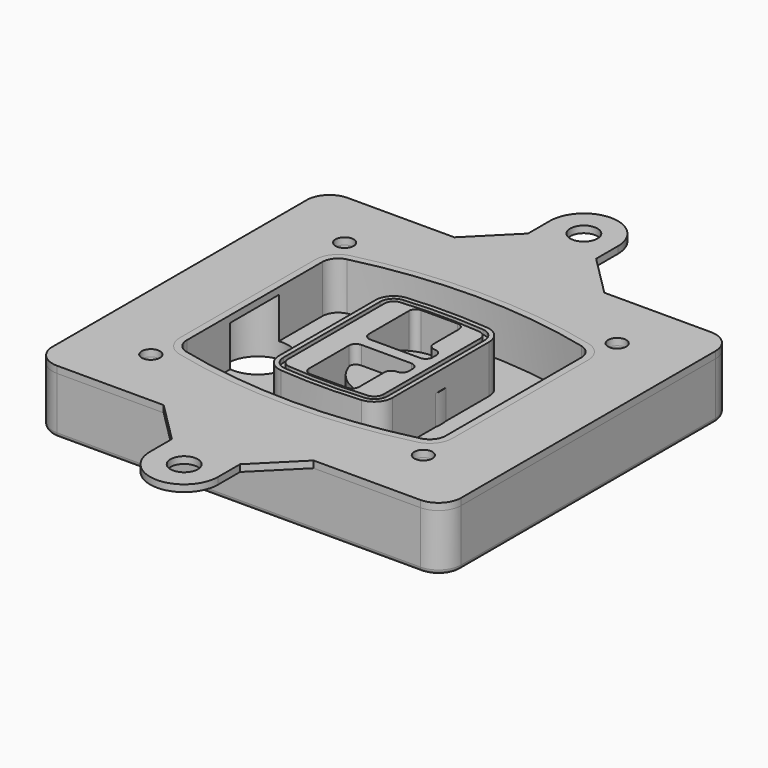
from build123d import *

# Parameters (mm, degrees)
F0_R      = 4
F1_DEPTH  = 25
F2_DEPTH  = 3
F3_DEPTH  = 18
F5_DEPTH  = 21
F6_DEPTH  = 2
F8_DEPTH  = 20
F9_DEPTH  = 16
F10_DEPTH = 25
F7_R      = 6
F7_R_2    = 4
F11_DEPTH = 6
F13_DEPTH = 9
F15_R     = 2
F16_R     = 4
F16_R_2   = 6
F17_DEPTH = 3


# Not quite as in the source:
# - a feature of the source that left no trace in its solid (it failed there, or was rolled back) is left out
# - a feature names something its author has since deleted; it is built from what else it names


with BuildPart() as f1:
    # F0 (on Top) → F1 (new body)
    with BuildSketch(Plane.XY):
        with BuildLine():
            ThreePointArc((-90, -70), (-87.0710678119, -77.0710678119), (-80, -80))
            Line((-80, -80), (80, -80))
            ThreePointArc((80, -80), (87.0710678119, -77.0710678119), (90, -70))
            Line((90, -70), (90, 70))
            ThreePointArc((90, 70), (87.0710678119, 77.0710678119), (80, 80))
            Line((80, 80), (-80, 80))
            ThreePointArc((-80, 80), (-87.0710678119, 77.0710678119), (-90, 70))
            Line((-90, 70), (-90, -70))
        make_face()
        with Locations((-60, -53.3333333333)):
            Circle(F0_R, mode=Mode.SUBTRACT)
        with Locations((60, -53.3333333333)):
            Circle(F0_R, mode=Mode.SUBTRACT)
        with Locations((-60, 53.3333333333)):
            Circle(F0_R, mode=Mode.SUBTRACT)
        with BuildLine():
            ThreePointArc((-64, 37.2990447398), (-61.0143011354, 45.9411029726), (-53.3306899286, 50.8970778549))
            ThreePointArc((-53.3306899286, 50.8970778549), (0, 57.3333333333), (53.3306899286, 50.8970778549))
            ThreePointArc((53.3306899286, 50.8970778549), (61.0143011354, 45.9411029726), (64, 37.2990447398))
            Line((64, 37.2990447398), (64, -37.2990447398))
            ThreePointArc((64, -37.2990447398), (61.0143011354, -45.9411029726), (53.3306899286, -50.8970778549))
            ThreePointArc((53.3306899286, -50.8970778549), (0, -57.3333333333), (-53.3306899286, -50.8970778549))
            ThreePointArc((-53.3306899286, -50.8970778549), (-61.0143011354, -45.9411029726), (-64, -37.2990447398))
            Line((-64, -37.2990447398), (-64, 37.2990447398))
        make_face(mode=Mode.SUBTRACT)
        with Locations((60, 53.3333333333)):
            Circle(F0_R, mode=Mode.SUBTRACT)
        with BuildLine():
            ThreePointArc((53.3306899286, 50.8970778549), (0, 57.3333333333), (-53.3306899286, 50.8970778549))
            ThreePointArc((-53.3306899286, 50.8970778549), (-61.0143011354, 45.9411029726), (-64, 37.2990447398))
            Line((-64, 37.2990447398), (-64, -37.2990447398))
            ThreePointArc((-64, -37.2990447398), (-61.0143011354, -45.9411029726), (-53.3306899286, -50.8970778549))
            ThreePointArc((-53.3306899286, -50.8970778549), (0, -57.3333333333), (53.3306899286, -50.8970778549))
            ThreePointArc((53.3306899286, -50.8970778549), (61.0143011354, -45.9411029726), (64, -37.2990447398))
            Line((64, -37.2990447398), (64, 37.2990447398))
            ThreePointArc((64, 37.2990447398), (61.0143011354, 45.9411029726), (53.3306899286, 50.8970778549))
        make_face()
        with BuildLine():
            Line((-60, -37.2990447398), (-60, 37.2990447398))
            ThreePointArc((-60, 37.2990447398), (-57.8673579538, 43.4719434775), (-52.3790642347, 47.0119255363))
            ThreePointArc((-52.3790642347, 47.0119255363), (0, 53.3333333333), (52.3790642347, 47.0119255363))
            ThreePointArc((52.3790642347, 47.0119255363), (57.8673579538, 43.4719434775), (60, 37.2990447398))
            Line((60, 37.2990447398), (60, -37.2990447398))
            ThreePointArc((60, -37.2990447398), (57.8673579538, -43.4719434775), (52.3790642347, -47.0119255363))
            ThreePointArc((52.3790642347, -47.0119255363), (0, -53.3333333333), (-52.3790642347, -47.0119255363))
            ThreePointArc((-52.3790642347, -47.0119255363), (-57.8673579538, -43.4719434775), (-60, -37.2990447398))
        make_face(mode=Mode.SUBTRACT)
        with BuildLine():
            ThreePointArc((-52.3790642347, 47.0119255363), (-57.8673579538, 43.4719434775), (-60, 37.2990447398))
            Line((-60, 37.2990447398), (-60, -37.2990447398))
            ThreePointArc((-60, -37.2990447398), (-57.8673579538, -43.4719434775), (-52.3790642347, -47.0119255363))
            ThreePointArc((-52.3790642347, -47.0119255363), (0, -53.3333333333), (52.3790642347, -47.0119255363))
            ThreePointArc((52.3790642347, -47.0119255363), (57.8673579538, -43.4719434775), (60, -37.2990447398))
            Line((60, -37.2990447398), (60, 37.2990447398))
            ThreePointArc((60, 37.2990447398), (57.8673579538, 43.4719434775), (52.3790642347, 47.0119255363))
            ThreePointArc((52.3790642347, 47.0119255363), (0, 53.3333333333), (-52.3790642347, 47.0119255363))
        make_face()
        with BuildLine():
            ThreePointArc((51.6653449643, 44.0980612973), (55.5071505677, 41.6200738562), (57, 37.2990447398))
            Line((57, 37.2990447398), (57, -37.2990447398))
            ThreePointArc((57, -37.2990447398), (55.5071505677, -41.6200738562), (51.6653449643, -44.0980612973))
            ThreePointArc((51.6653449643, -44.0980612973), (0, -50.3333333333), (-51.6653449643, -44.0980612973))
            ThreePointArc((-51.6653449643, -44.0980612973), (-55.5071505677, -41.6200738562), (-57, -37.2990447398))
            Line((-57, -37.2990447398), (-57, 37.2990447398))
            ThreePointArc((-57, 37.2990447398), (-55.5071505677, 41.6200738562), (-51.6653449643, 44.0980612973))
            ThreePointArc((-51.6653449643, 44.0980612973), (0, 50.3333333333), (51.6653449643, 44.0980612973))
        make_face(mode=Mode.SUBTRACT)
        with BuildLine():
            Line((57, -37.2990447398), (57, 37.2990447398))
            ThreePointArc((57, 37.2990447398), (55.5071505677, 41.6200738562), (51.6653449643, 44.0980612973))
            ThreePointArc((51.6653449643, 44.0980612973), (0, 50.3333333333), (-51.6653449643, 44.0980612973))
            ThreePointArc((-51.6653449643, 44.0980612973), (-55.5071505677, 41.6200738562), (-57, 37.2990447398))
            Line((-57, 37.2990447398), (-57, -37.2990447398))
            ThreePointArc((-57, -37.2990447398), (-55.5071505677, -41.6200738562), (-51.6653449643, -44.0980612973))
            ThreePointArc((-51.6653449643, -44.0980612973), (0, -50.3333333333), (51.6653449643, -44.0980612973))
            ThreePointArc((51.6653449643, -44.0980612973), (55.5071505677, -41.6200738562), (57, -37.2990447398))
        make_face()
    extrude(amount=-F1_DEPTH)

    # F0 (on Top) → F2 (join)
    with BuildSketch(Plane.XY):
        with BuildLine():
            ThreePointArc((-52.3790642347, 47.0119255363), (-57.8673579538, 43.4719434775), (-60, 37.2990447398))
            Line((-60, 37.2990447398), (-60, -37.2990447398))
            ThreePointArc((-60, -37.2990447398), (-57.8673579538, -43.4719434775), (-52.3790642347, -47.0119255363))
            ThreePointArc((-52.3790642347, -47.0119255363), (0, -53.3333333333), (52.3790642347, -47.0119255363))
            ThreePointArc((52.3790642347, -47.0119255363), (57.8673579538, -43.4719434775), (60, -37.2990447398))
            Line((60, -37.2990447398), (60, 37.2990447398))
            ThreePointArc((60, 37.2990447398), (57.8673579538, 43.4719434775), (52.3790642347, 47.0119255363))
            ThreePointArc((52.3790642347, 47.0119255363), (0, 53.3333333333), (-52.3790642347, 47.0119255363))
        make_face()
        with BuildLine():
            ThreePointArc((51.6653449643, 44.0980612973), (55.5071505677, 41.6200738562), (57, 37.2990447398))
            Line((57, 37.2990447398), (57, -37.2990447398))
            ThreePointArc((57, -37.2990447398), (55.5071505677, -41.6200738562), (51.6653449643, -44.0980612973))
            ThreePointArc((51.6653449643, -44.0980612973), (0, -50.3333333333), (-51.6653449643, -44.0980612973))
            ThreePointArc((-51.6653449643, -44.0980612973), (-55.5071505677, -41.6200738562), (-57, -37.2990447398))
            Line((-57, -37.2990447398), (-57, 37.2990447398))
            ThreePointArc((-57, 37.2990447398), (-55.5071505677, 41.6200738562), (-51.6653449643, 44.0980612973))
            ThreePointArc((-51.6653449643, 44.0980612973), (0, 50.3333333333), (51.6653449643, 44.0980612973))
        make_face(mode=Mode.SUBTRACT)
    extrude(amount=F2_DEPTH)

    # F0 (on Top) → F3 (cut)
    with BuildSketch(Plane.XY):
        with BuildLine():
            Line((57, -37.2990447398), (57, 37.2990447398))
            ThreePointArc((57, 37.2990447398), (55.5071505677, 41.6200738562), (51.6653449643, 44.0980612973))
            ThreePointArc((51.6653449643, 44.0980612973), (0, 50.3333333333), (-51.6653449643, 44.0980612973))
            ThreePointArc((-51.6653449643, 44.0980612973), (-55.5071505677, 41.6200738562), (-57, 37.2990447398))
            Line((-57, 37.2990447398), (-57, -37.2990447398))
            ThreePointArc((-57, -37.2990447398), (-55.5071505677, -41.6200738562), (-51.6653449643, -44.0980612973))
            ThreePointArc((-51.6653449643, -44.0980612973), (0, -50.3333333333), (51.6653449643, -44.0980612973))
            ThreePointArc((51.6653449643, -44.0980612973), (55.5071505677, -41.6200738562), (57, -37.2990447398))
        make_face()
    extrude(amount=-F3_DEPTH, mode=Mode.SUBTRACT)

    # F4 (on face) → F5 (join, through all)
    with BuildSketch(Plane.XY.offset(3)):
        with BuildLine():
            ThreePointArc((-25, -26.587695628), (-22.8992979869, -31.9912392117), (-17.7004291845, -34.5569740744))
            ThreePointArc((-17.7004291845, -34.5569740744), (0, -35.3333333333), (17.7004291845, -34.5569740744))
            ThreePointArc((17.7004291845, -34.5569740744), (22.8992979869, -31.9912392117), (25, -26.587695628))
            Line((25, -26.587695628), (25, 26.587695628))
            ThreePointArc((25, 26.587695628), (22.8992979869, 31.9912392117), (17.7004291845, 34.5569740744))
            ThreePointArc((17.7004291845, 34.5569740744), (0, 35.3333333333), (-17.7004291845, 34.5569740744))
            ThreePointArc((-17.7004291845, 34.5569740744), (-22.8992979869, 31.9912392117), (-25, 26.587695628))
            Line((-25, 26.587695628), (-25, -26.587695628))
        make_face()
        with BuildLine():
            ThreePointArc((17.5253218884, 32.5646544628), (21.4244734902, 30.6403533158), (23, 26.587695628))
            Line((23, 26.587695628), (23, -26.587695628))
            ThreePointArc((23, -26.587695628), (21.4244734902, -30.6403533158), (17.5253218884, -32.5646544628))
            ThreePointArc((17.5253218884, -32.5646544628), (0, -33.3333333333), (-17.5253218884, -32.5646544628))
            ThreePointArc((-17.5253218884, -32.5646544628), (-21.4244734902, -30.6403533158), (-23, -26.587695628))
            Line((-23, -26.587695628), (-23, 26.587695628))
            ThreePointArc((-23, 26.587695628), (-21.4244734902, 30.6403533158), (-17.5253218884, 32.5646544628))
            ThreePointArc((-17.5253218884, 32.5646544628), (0, 33.3333333333), (17.5253218884, 32.5646544628))
        make_face(mode=Mode.SUBTRACT)
        with BuildLine():
            Line((23, -26.587695628), (23, 26.587695628))
            ThreePointArc((23, 26.587695628), (21.4244734902, 30.6403533158), (17.5253218884, 32.5646544628))
            ThreePointArc((17.5253218884, 32.5646544628), (0, 33.3333333333), (-17.5253218884, 32.5646544628))
            ThreePointArc((-17.5253218884, 32.5646544628), (-21.4244734902, 30.6403533158), (-23, 26.587695628))
            Line((-23, 26.587695628), (-23, -26.587695628))
            ThreePointArc((-23, -26.587695628), (-21.4244734902, -30.6403533158), (-17.5253218884, -32.5646544628))
            ThreePointArc((-17.5253218884, -32.5646544628), (0, -33.3333333333), (17.5253218884, -32.5646544628))
            ThreePointArc((17.5253218884, -32.5646544628), (21.4244734902, -30.6403533158), (23, -26.587695628))
        make_face()
        with BuildLine():
            ThreePointArc((17.3502145923, 30.5723348512), (19.9496489934, 29.2894674198), (21, 26.587695628))
            Line((21, 26.587695628), (21, -26.587695628))
            ThreePointArc((21, -26.587695628), (19.9496489934, -29.2894674198), (17.3502145923, -30.5723348512))
            ThreePointArc((17.3502145923, -30.5723348512), (0, -31.3333333333), (-17.3502145923, -30.5723348512))
            ThreePointArc((-17.3502145923, -30.5723348512), (-19.9496489934, -29.2894674198), (-21, -26.587695628))
            Line((-21, -26.587695628), (-21, 26.587695628))
            ThreePointArc((-21, 26.587695628), (-19.9496489934, 29.2894674198), (-17.3502145923, 30.5723348512))
            ThreePointArc((-17.3502145923, 30.5723348512), (0, 31.3333333333), (17.3502145923, 30.5723348512))
        make_face(mode=Mode.SUBTRACT)
        with BuildLine():
            Line((21, -26.587695628), (21, 26.587695628))
            ThreePointArc((21, 26.587695628), (19.9496489934, 29.2894674198), (17.3502145923, 30.5723348512))
            ThreePointArc((17.3502145923, 30.5723348512), (0, 31.3333333333), (-17.3502145923, 30.5723348512))
            ThreePointArc((-17.3502145923, 30.5723348512), (-19.9496489934, 29.2894674198), (-21, 26.587695628))
            Line((-21, 26.587695628), (-21, -26.587695628))
            ThreePointArc((-21, -26.587695628), (-19.9496489934, -29.2894674198), (-17.3502145923, -30.5723348512))
            ThreePointArc((-17.3502145923, -30.5723348512), (0, -31.3333333333), (17.3502145923, -30.5723348512))
            ThreePointArc((17.3502145923, -30.5723348512), (19.9496489934, -29.2894674198), (21, -26.587695628))
        make_face()
        with BuildLine():
            Line((-8, -2.5), (14, -2.5))
            ThreePointArc((14, -2.5), (16.1213203436, -3.3786796564), (17, -5.5))
            Line((17, -5.5), (17, -7.5))
            ThreePointArc((17, -7.5), (16.1213203436, -9.6213203436), (14, -10.5))
            ThreePointArc((14, -10.5), (11.8786796564, -11.3786796564), (11, -13.5))
            Line((11, -13.5), (11, -27.5))
            ThreePointArc((11, -27.5), (10.1213203436, -29.6213203436), (8, -30.5))
            Line((8, -30.5), (-8, -30.5))
            ThreePointArc((-8, -30.5), (-10.1213203436, -29.6213203436), (-11, -27.5))
            Line((-11, -27.5), (-11, -5.5))
            ThreePointArc((-11, -5.5), (-10.1213203436, -3.3786796564), (-8, -2.5))
        make_face(mode=Mode.SUBTRACT)
        with BuildLine():
            ThreePointArc((-8, 2.5), (-10.1213203436, 3.3786796564), (-11, 5.5))
            Line((-11, 5.5), (-11, 27.5))
            ThreePointArc((-11, 27.5), (-10.1213203436, 29.6213203436), (-8, 30.5))
            Line((-8, 30.5), (8, 30.5))
            ThreePointArc((8, 30.5), (10.1213203436, 29.6213203436), (11, 27.5))
            Line((11, 27.5), (11, 13.5))
            ThreePointArc((11, 13.5), (11.8786796564, 11.3786796564), (14, 10.5))
            ThreePointArc((14, 10.5), (16.1213203436, 9.6213203436), (17, 7.5))
            Line((17, 7.5), (17, 5.5))
            ThreePointArc((17, 5.5), (16.1213203436, 3.3786796564), (14, 2.5))
            Line((14, 2.5), (-8, 2.5))
        make_face(mode=Mode.SUBTRACT)
    extrude(amount=-F5_DEPTH)

    # F4 (on face) → F6 (cut)
    with BuildSketch(Plane.XY.offset(3)):
        with BuildLine():
            Line((23, -26.587695628), (23, 26.587695628))
            ThreePointArc((23, 26.587695628), (21.4244734902, 30.6403533158), (17.5253218884, 32.5646544628))
            ThreePointArc((17.5253218884, 32.5646544628), (0, 33.3333333333), (-17.5253218884, 32.5646544628))
            ThreePointArc((-17.5253218884, 32.5646544628), (-21.4244734902, 30.6403533158), (-23, 26.587695628))
            Line((-23, 26.587695628), (-23, -26.587695628))
            ThreePointArc((-23, -26.587695628), (-21.4244734902, -30.6403533158), (-17.5253218884, -32.5646544628))
            ThreePointArc((-17.5253218884, -32.5646544628), (0, -33.3333333333), (17.5253218884, -32.5646544628))
            ThreePointArc((17.5253218884, -32.5646544628), (21.4244734902, -30.6403533158), (23, -26.587695628))
        make_face()
        with BuildLine():
            ThreePointArc((17.3502145923, 30.5723348512), (19.9496489934, 29.2894674198), (21, 26.587695628))
            Line((21, 26.587695628), (21, -26.587695628))
            ThreePointArc((21, -26.587695628), (19.9496489934, -29.2894674198), (17.3502145923, -30.5723348512))
            ThreePointArc((17.3502145923, -30.5723348512), (0, -31.3333333333), (-17.3502145923, -30.5723348512))
            ThreePointArc((-17.3502145923, -30.5723348512), (-19.9496489934, -29.2894674198), (-21, -26.587695628))
            Line((-21, -26.587695628), (-21, 26.587695628))
            ThreePointArc((-21, 26.587695628), (-19.9496489934, 29.2894674198), (-17.3502145923, 30.5723348512))
            ThreePointArc((-17.3502145923, 30.5723348512), (0, 31.3333333333), (17.3502145923, 30.5723348512))
        make_face(mode=Mode.SUBTRACT)
    extrude(amount=-F6_DEPTH, mode=Mode.SUBTRACT)

    # F7 (on face) → F8 (join)
    with BuildSketch(Plane(origin=(0, 0, -25), x_dir=(1, 0, 0), z_dir=(0, 0, -1))):
        with BuildLine():
            ThreePointArc((-6.71157564, 0), (6.7567035675, 13.4682792075), (20.224982775, 0))
            Line((20.224982775, 0), (25.224982775, 0))
            ThreePointArc((25.224982775, 0), (6.7567035675, 18.4682792075), (-11.71157564, 0))
            Line((-11.71157564, 0), (-6.71157564, 0))
        make_face()
        with BuildLine():
            Line((-6.71157564, 0), (20.224982775, 0))
            ThreePointArc((20.224982775, 0), (6.7567035675, 13.4682792075), (-6.71157564, 0))
        make_face()
        with BuildLine():
            ThreePointArc((-6.71157564, 0), (6.7567035675, -13.4682792075), (20.224982775, 0))
            Line((20.224982775, 0), (-6.71157564, 0))
        make_face()
        with BuildLine():
            Line((25.224982775, 0), (20.224982775, 0))
            ThreePointArc((20.224982775, 0), (6.7567035675, -13.4682792075), (-6.71157564, 0))
            Line((-6.71157564, 0), (-11.71157564, 0))
            ThreePointArc((-11.71157564, 0), (6.7567035675, -18.4682792075), (25.224982775, 0))
        make_face()
    extrude(amount=-F8_DEPTH)

    # F7 (on face) → F9 (cut)
    with BuildSketch(Plane(origin=(0, 0, -25), x_dir=(1, 0, 0), z_dir=(0, 0, -1))):
        with BuildLine():
            Line((-6.71157564, 0), (20.224982775, 0))
            ThreePointArc((20.224982775, 0), (6.7567035675, 13.4682792075), (-6.71157564, 0))
        make_face()
        with BuildLine():
            ThreePointArc((-6.71157564, 0), (6.7567035675, -13.4682792075), (20.224982775, 0))
            Line((20.224982775, 0), (-6.71157564, 0))
        make_face()
    extrude(amount=-F9_DEPTH, mode=Mode.SUBTRACT)

    # F7 (on face) → F10 (cut)
    with BuildSketch(Plane(origin=(0, 0, -25), x_dir=(1, 0, 0), z_dir=(0, 0, -1))):
        with BuildLine():
            Line((-69.0318229325, 0), (-42.0952645175, 0))
            ThreePointArc((-42.0952645175, 0), (-55.563543725, 13.4682792075), (-69.0318229325, 0))
        make_face()
        with BuildLine():
            ThreePointArc((-69.0318229325, 0), (-55.563543725, -13.4682792075), (-42.0952645175, 0))
            Line((-42.0952645175, 0), (-69.0318229325, 0))
        make_face()
    extrude(amount=-F10_DEPTH, mode=Mode.SUBTRACT)

    # F7 (on face) → F11 (cut)
    with BuildSketch(Plane(origin=(0, 0, -25), x_dir=(1, 0, 0), z_dir=(0, 0, -1))):
        with Locations((60, -53.3333333333)):
            Circle(F7_R)
        with Locations((60, -53.3333333333)):
            Circle(F7_R_2, mode=Mode.SUBTRACT)
        with Locations((-60, -53.3333333333)):
            Circle(F7_R)
        with Locations((-60, -53.3333333333)):
            Circle(F7_R_2, mode=Mode.SUBTRACT)
        with Locations((-60, 53.3333333333)):
            Circle(F7_R)
        with Locations((-60, 53.3333333333)):
            Circle(F7_R_2, mode=Mode.SUBTRACT)
        with Locations((60, 53.3333333333)):
            Circle(F7_R)
        with Locations((60, 53.3333333333)):
            Circle(F7_R_2, mode=Mode.SUBTRACT)
    extrude(amount=-F11_DEPTH, mode=Mode.SUBTRACT)

    # F12 (on face) → F13 (cut, through all)
    with BuildSketch(Plane(origin=(0, 0, -9), x_dir=(1, 0, 0), z_dir=(0, 0, -1))):
        with BuildLine():
            ThreePointArc((20.224982775, 0), (20.1663399806, 1.2554664788), (19.9909222755, 2.5))
            Line((19.9909222755, 2.5), (14, 2.5))
            ThreePointArc((14, 2.5), (16.1213203436, 3.3786796564), (17, 5.5))
            Line((17, 5.5), (17, 7.5))
            ThreePointArc((17, 7.5), (16.1213203436, 9.6213203436), (14, 10.5))
            ThreePointArc((14, 10.5), (12.1627255951, 11.1284134507), (11.0951631559, 12.750384826))
            ThreePointArc((11.0951631559, 12.750384826), (11.0476113807, 12.7664660322), (11, 12.7823698976))
            Line((11, 12.7823698976), (11, -12.7823698976))
            ThreePointArc((11, -12.7823698976), (11.0476113807, -12.7664660322), (11.0951631559, -12.750384826))
            ThreePointArc((11.0951631559, -12.750384826), (12.1627255951, -11.1284134507), (14, -10.5))
            ThreePointArc((14, -10.5), (16.1213203436, -9.6213203436), (17, -7.5))
            Line((17, -7.5), (17, -5.5))
            ThreePointArc((17, -5.5), (16.1213203436, -3.3786796564), (14, -2.5))
            Line((14, -2.5), (19.9909222755, -2.5))
            ThreePointArc((19.9909222755, -2.5), (20.1663399806, -1.2554664788), (20.224982775, 0))
        make_face()
    extrude(amount=F13_DEPTH, mode=Mode.SUBTRACT)

    # F15
    f15_edges = [f1.edges().sort_by_distance(p)[0] for p in [
        (0, -80, -25),
        (-87.071068, -77.071068, -25),
        (-90, 0, -25),
        (-87.071068, 77.071068, -25),
        (87.071068, -77.071068, -25),
        (0, 80, -25),
        (90, 0, -25),
        (87.071068, 77.071068, -25),
    ]]
    fillet(f15_edges, radius=F15_R)


with BuildPart() as f17:
    # F16 (on face) → F17 (new body, through all)
    with BuildSketch(Plane.XY):
        with BuildLine():
            Line((-33, 80), (-80, 80))
            ThreePointArc((-80, 80), (-87.0710678119, 77.0710678119), (-90, 70))
            Line((-90, 70), (-90, -70))
            ThreePointArc((-90, -70), (-87.0710678119, -77.0710678119), (-80, -80))
            Line((-80, -80), (-33, -80))
            Line((-33, -80), (33, -80))
            Line((33, -80), (80, -80))
            ThreePointArc((80, -80), (87.0710678119, -77.0710678119), (90, -70))
            Line((90, -70), (90, 70))
            ThreePointArc((90, 70), (87.0710678119, 77.0710678119), (80, 80))
            Line((80, 80), (33, 80))
            Line((33, 80), (-33, 80))
        make_face()
        with Locations((-60, -53.3333333333)):
            Circle(F16_R, mode=Mode.SUBTRACT)
        with Locations((60, -53.3333333333)):
            Circle(F16_R, mode=Mode.SUBTRACT)
        with Locations((-60, 53.3333333333)):
            Circle(F16_R, mode=Mode.SUBTRACT)
        with BuildLine():
            ThreePointArc((52.3790642347, -47.0119255363), (0, -53.3333333333), (-52.3790642347, -47.0119255363))
            ThreePointArc((-52.3790642347, -47.0119255363), (-57.8673579538, -43.4719434775), (-60, -37.2990447398))
            Line((-60, -37.2990447398), (-60, 37.2990447398))
            ThreePointArc((-60, 37.2990447398), (-57.8673579538, 43.4719434775), (-52.3790642347, 47.0119255363))
            ThreePointArc((-52.3790642347, 47.0119255363), (0, 53.3333333333), (52.3790642347, 47.0119255363))
            ThreePointArc((52.3790642347, 47.0119255363), (57.8673579538, 43.4719434775), (60, 37.2990447398))
            Line((60, 37.2990447398), (60, -37.2990447398))
            ThreePointArc((60, -37.2990447398), (57.8673579538, -43.4719434775), (52.3790642347, -47.0119255363))
        make_face(mode=Mode.SUBTRACT)
        with Locations((60, 53.3333333333)):
            Circle(F16_R, mode=Mode.SUBTRACT)
        with BuildLine():
            Line((-15, 98), (-33, 80))
            Line((-33, 80), (33, 80))
            Line((33, 80), (15, 98))
            Line((15, 98), (15, 110))
            ThreePointArc((15, 110), (0, 125), (-15, 110))
            Line((-15, 110), (-15, 98))
        make_face()
        with Locations((0, 110)):
            Circle(F16_R_2, mode=Mode.SUBTRACT)
        with BuildLine():
            Line((33, -80), (-33, -80))
            Line((-33, -80), (-15, -98))
            Line((-15, -98), (-15, -110))
            ThreePointArc((-15, -110), (0, -125), (15, -110))
            Line((15, -110), (15, -98))
            Line((15, -98), (33, -80))
        make_face()
        with Locations((0, -110)):
            Circle(F16_R_2, mode=Mode.SUBTRACT)
    extrude(amount=F17_DEPTH)


solid = Compound([f1.part, f17.part])
